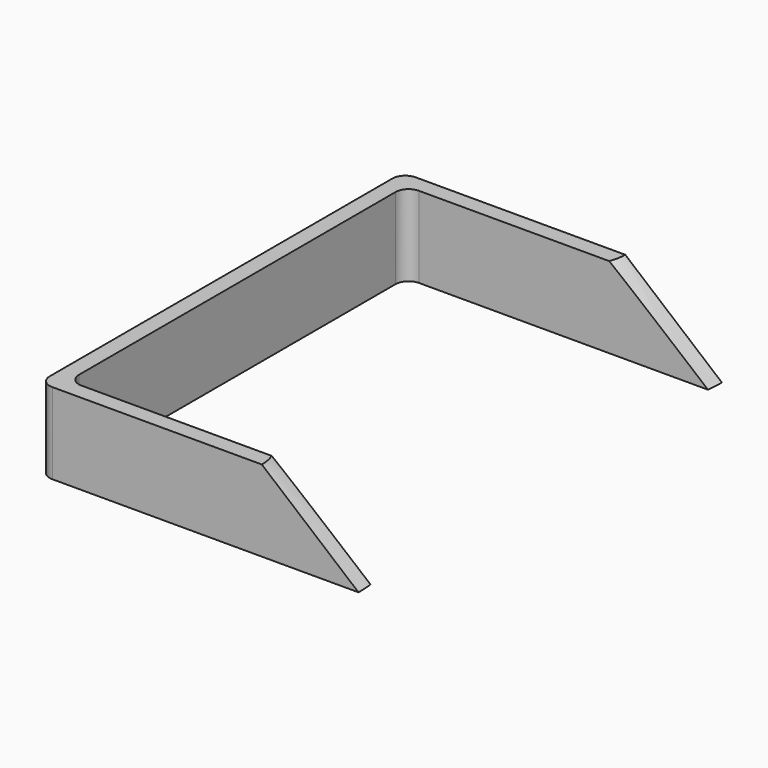
from build123d import *

# Parameters (mm, degrees)
F1_DEPTH     = 3.175
F2_DEPTH     = 19.05
F3_DEPTH     = 3.175
F4_T4_ANGLE  = 359.64
F4_T11_ANGLE = 359.64
F4_T16_ANGLE = 359.64
F4_T18_ANGLE = 359.64
F5_R         = 2.54
F6_W         = 173.444584012
F6_H         = 315.2023479342
F7_DEPTH     = 3.175


# Not quite as in the source:
# - a fillet or chamfer that OpenCascade refuses, or shapes differently, is made with other operations: its cross-section is extruded or revolved along the edge and cut away or added


with BuildPart() as f1:
    # F0 (on Top) → F1 (new body)
    with BuildSketch(Plane.XY):
        with BuildLine():
            Line((-34.925, 44.45), (-28.575, 44.45))
            ThreePointArc((-28.575, 44.45), (-39.4151280605, 48.9401280605), (-34.925, 38.1))
            Line((-34.925, 38.1), (-34.925, 44.45))
        make_face()
        with BuildLine():
            ThreePointArc((6.35, 44.45), (0, 50.8), (-6.35, 44.45))
            Line((-6.35, 44.45), (6.35, 44.45))
        make_face()
        with BuildLine():
            Line((-34.925, -44.45), (-34.925, -38.1))
            ThreePointArc((-34.925, -38.1), (-39.4151280605, -48.9401280605), (-28.575, -44.45))
            Line((-28.575, -44.45), (-34.925, -44.45))
        make_face()
        with BuildLine():
            Line((6.35, -44.45), (-6.35, -44.45))
            ThreePointArc((-6.35, -44.45), (0, -50.8), (6.35, -44.45))
        make_face()
        with BuildLine():
            ThreePointArc((-28.575, 44.45), (-28.7913710031, 42.8064990636), (-29.425738686, 41.275))
            Line((-29.425738686, 41.275), (-5.499261314, 41.275))
            ThreePointArc((-5.499261314, 41.275), (-6.1336289969, 42.8064990636), (-6.35, 44.45))
            Line((-6.35, 44.45), (-28.575, 44.45))
        make_face()
        with BuildLine():
            Line((-5.499261314, -41.275), (-29.425738686, -41.275))
            ThreePointArc((-29.425738686, -41.275), (-28.7913710031, -42.8064990636), (-28.575, -44.45))
            Line((-28.575, -44.45), (-6.35, -44.45))
            ThreePointArc((-6.35, -44.45), (-6.1336289969, -42.8064990636), (-5.499261314, -41.275))
        make_face()
        with BuildLine():
            Line((-31.75, -38.950738686), (-31.75, 38.950738686))
            ThreePointArc((-31.75, 38.950738686), (-33.2814990636, 38.3163710031), (-34.925, 38.1))
            Line((-34.925, 38.1), (-34.925, -38.1))
            ThreePointArc((-34.925, -38.1), (-33.2814990636, -38.3163710031), (-31.75, -38.950738686))
        make_face()
        with BuildLine():
            Line((-31.75, 38.950738686), (-31.75, 41.275))
            Line((-31.75, 41.275), (-29.425738686, 41.275))
            ThreePointArc((-29.425738686, 41.275), (-28.7913710031, 42.8064990636), (-28.575, 44.45))
            Line((-28.575, 44.45), (-34.925, 44.45))
            Line((-34.925, 44.45), (-34.925, 38.1))
            ThreePointArc((-34.925, 38.1), (-33.2814990636, 38.3163710031), (-31.75, 38.950738686))
        make_face()
        with BuildLine():
            ThreePointArc((-6.35, 44.45), (-6.1336289969, 42.8064990636), (-5.499261314, 41.275))
            Line((-5.499261314, 41.275), (5.499261314, 41.275))
            ThreePointArc((5.499261314, 41.275), (6.1336289969, 42.8064990636), (6.35, 44.45))
            Line((6.35, 44.45), (-6.35, 44.45))
        make_face()
        with BuildLine():
            Line((-31.75, -41.275), (-31.75, -38.950738686))
            ThreePointArc((-31.75, -38.950738686), (-33.2814990636, -38.3163710031), (-34.925, -38.1))
            Line((-34.925, -38.1), (-34.925, -44.45))
            Line((-34.925, -44.45), (-28.575, -44.45))
            ThreePointArc((-28.575, -44.45), (-28.7913710031, -42.8064990636), (-29.425738686, -41.275))
            Line((-29.425738686, -41.275), (-31.75, -41.275))
        make_face()
        with BuildLine():
            Line((5.499261314, -41.275), (-5.499261314, -41.275))
            ThreePointArc((-5.499261314, -41.275), (-6.1336289969, -42.8064990636), (-6.35, -44.45))
            Line((-6.35, -44.45), (6.35, -44.45))
            ThreePointArc((6.35, -44.45), (6.1336289969, -42.8064990636), (5.499261314, -41.275))
        make_face()
    extrude(amount=F1_DEPTH)

    # F0 (on Top) → F2 (join)
    with BuildSketch(Plane.XY):
        with BuildLine():
            ThreePointArc((-28.575, 44.45), (-28.7913710031, 42.8064990636), (-29.425738686, 41.275))
            Line((-29.425738686, 41.275), (-5.499261314, 41.275))
            ThreePointArc((-5.499261314, 41.275), (-6.1336289969, 42.8064990636), (-6.35, 44.45))
            Line((-6.35, 44.45), (-28.575, 44.45))
        make_face()
        with BuildLine():
            ThreePointArc((-6.35, 44.45), (-6.1336289969, 42.8064990636), (-5.499261314, 41.275))
            Line((-5.499261314, 41.275), (5.499261314, 41.275))
            ThreePointArc((5.499261314, 41.275), (6.1336289969, 42.8064990636), (6.35, 44.45))
            Line((6.35, 44.45), (-6.35, 44.45))
        make_face()
        with BuildLine():
            Line((-31.75, 38.950738686), (-31.75, 41.275))
            Line((-31.75, 41.275), (-29.425738686, 41.275))
            ThreePointArc((-29.425738686, 41.275), (-28.7913710031, 42.8064990636), (-28.575, 44.45))
            Line((-28.575, 44.45), (-34.925, 44.45))
            Line((-34.925, 44.45), (-34.925, 38.1))
            ThreePointArc((-34.925, 38.1), (-33.2814990636, 38.3163710031), (-31.75, 38.950738686))
        make_face()
        with BuildLine():
            Line((-31.75, -38.950738686), (-31.75, 38.950738686))
            ThreePointArc((-31.75, 38.950738686), (-33.2814990636, 38.3163710031), (-34.925, 38.1))
            Line((-34.925, 38.1), (-34.925, -38.1))
            ThreePointArc((-34.925, -38.1), (-33.2814990636, -38.3163710031), (-31.75, -38.950738686))
        make_face()
        with BuildLine():
            Line((-31.75, -41.275), (-31.75, -38.950738686))
            ThreePointArc((-31.75, -38.950738686), (-33.2814990636, -38.3163710031), (-34.925, -38.1))
            Line((-34.925, -38.1), (-34.925, -44.45))
            Line((-34.925, -44.45), (-28.575, -44.45))
            ThreePointArc((-28.575, -44.45), (-28.7913710031, -42.8064990636), (-29.425738686, -41.275))
            Line((-29.425738686, -41.275), (-31.75, -41.275))
        make_face()
        with BuildLine():
            Line((-5.499261314, -41.275), (-29.425738686, -41.275))
            ThreePointArc((-29.425738686, -41.275), (-28.7913710031, -42.8064990636), (-28.575, -44.45))
            Line((-28.575, -44.45), (-6.35, -44.45))
            ThreePointArc((-6.35, -44.45), (-6.1336289969, -42.8064990636), (-5.499261314, -41.275))
        make_face()
        with BuildLine():
            Line((5.499261314, -41.275), (-5.499261314, -41.275))
            ThreePointArc((-5.499261314, -41.275), (-6.1336289969, -42.8064990636), (-6.35, -44.45))
            Line((-6.35, -44.45), (6.35, -44.45))
            ThreePointArc((6.35, -44.45), (6.1336289969, -42.8064990636), (5.499261314, -41.275))
        make_face()
    extrude(amount=F2_DEPTH)

    # F0 (on Top) → F3 (join)
    with BuildSketch(Plane.XY):
        with BuildLine():
            ThreePointArc((6.35, 44.45), (6.1336289969, 42.8064990636), (5.499261314, 41.275))
            Line((5.499261314, 41.275), (31.75, 41.275))
            Line((31.75, 41.275), (31.75, -41.275))
            Line((31.75, -41.275), (5.499261314, -41.275))
            ThreePointArc((5.499261314, -41.275), (6.1336289969, -42.8064990636), (6.35, -44.45))
            Line((6.35, -44.45), (34.925, -44.45))
            Line((34.925, -44.45), (34.925, 44.45))
            Line((34.925, 44.45), (6.35, 44.45))
        make_face()
        with BuildLine():
            Line((-5.499261314, 41.275), (-29.425738686, 41.275))
            ThreePointArc((-29.425738686, 41.275), (-30.4348719395, 39.9598719395), (-31.75, 38.950738686))
            Line((-31.75, 38.950738686), (-31.75, -38.950738686))
            ThreePointArc((-31.75, -38.950738686), (-30.4348719395, -39.9598719395), (-29.425738686, -41.275))
            Line((-29.425738686, -41.275), (-5.499261314, -41.275))
            ThreePointArc((-5.499261314, -41.275), (0, -38.1), (5.499261314, -41.275))
            Line((5.499261314, -41.275), (31.75, -41.275))
            Line((31.75, -41.275), (31.75, 41.275))
            Line((31.75, 41.275), (5.499261314, 41.275))
            ThreePointArc((5.499261314, 41.275), (0, 38.1), (-5.499261314, 41.275))
        make_face()
        with BuildLine():
            Line((5.499261314, 41.275), (-5.499261314, 41.275))
            ThreePointArc((-5.499261314, 41.275), (0, 38.1), (5.499261314, 41.275))
        make_face()
        with BuildLine():
            Line((-29.425738686, 41.275), (-31.75, 41.275))
            Line((-31.75, 41.275), (-31.75, 38.950738686))
            ThreePointArc((-31.75, 38.950738686), (-30.4348719395, 39.9598719395), (-29.425738686, 41.275))
        make_face()
        with BuildLine():
            ThreePointArc((5.499261314, -41.275), (0, -38.1), (-5.499261314, -41.275))
            Line((-5.499261314, -41.275), (5.499261314, -41.275))
        make_face()
        with BuildLine():
            ThreePointArc((-29.425738686, -41.275), (-30.4348719395, -39.9598719395), (-31.75, -38.950738686))
            Line((-31.75, -38.950738686), (-31.75, -41.275))
            Line((-31.75, -41.275), (-29.425738686, -41.275))
        make_face()
    extrude(amount=F3_DEPTH)

    # F4: chamfer of 17.78 x 21.1893788763 on 4 edges, made by hand


with BuildPart() as f4_tool2:
    # F4_s3 → F4_t4 (revolve)
    with BuildSketch(Plane(origin=(-7.9045602021, -1.4531788711, 0), x_dir=(0, 0, 1), z_dir=(-0.983517952, -0.1808105031, 0))):
        Polygon((3.175, -16.1779940912), (20.955, -37.3673729675), (3.175, -37.3673729675), align=None)
    revolve(axis=Axis((0, -44.45, 3.175), (0, 0, -1)), revolution_arc=F4_T4_ANGLE)

    split(bisect_by=Plane.XY.offset(19.05), keep=Keep.BOTTOM)

    split(bisect_by=Plane.XZ.offset(44.45), keep=Keep.BOTTOM)

    split(bisect_by=Plane.XZ.offset(41.275), keep=Keep.TOP)


with BuildPart() as f1_1:
    add(f1.part)

    # F4_t1: union F4_tool2
    add(f4_tool2.part)


with BuildPart() as f4_tool9:
    # F4_s10 → F4_t11 (revolve)
    with BuildSketch(Plane(origin=(-8.164955624, 1.5541479455, 0), x_dir=(0, 0, 1), z_dir=(0.9823624798, -0.186986519, 0))):
        Polygon((20.955, -37.3160122271), (3.175, -16.1266333508), (3.175, -37.3160122271), align=None)
    revolve(axis=Axis((0, 44.45, 3.175), (0, 0, -1)), revolution_arc=F4_T11_ANGLE)

    split(bisect_by=Plane.XZ.offset(-44.45), keep=Keep.TOP)

    split(bisect_by=Plane.XY.offset(19.05), keep=Keep.BOTTOM)

    split(bisect_by=Plane.XZ.offset(-41.275), keep=Keep.BOTTOM)


with BuildPart() as f1_2:
    add(f1_1.part)

    # F4_t8: union F4_tool9
    add(f4_tool9.part)

    # F4_s15 → F4_t16 (revolve, cut)
    with BuildSketch(Plane(origin=(-0.1396428746, -0.0004387025, 0), x_dir=(0, 0, 1), z_dir=(0.9999950652, 0.0031415875, 0))):
        Polygon((-14.605, 38.0997806482), (-9.276717342, 44.4497806482), (3.175, 44.4497806482), (3.175, 38.0997806482), align=None)
    revolve(axis=Axis((0, -44.45, 3.175), (0, 0, 1)), revolution_arc=F4_T16_ANGLE, mode=Mode.SUBTRACT)

    # F4_s17 → F4_t18 (revolve, cut)
    with BuildSketch(Plane(origin=(0.1396428746, 0.0004387025, 0), x_dir=(0, 0, 1), z_dir=(-0.9999950652, -0.0031415875, 0))):
        Polygon((-14.605, 38.0997806482), (-9.276717342, 44.4497806482), (3.175, 44.4497806482), (3.175, 38.0997806482), align=None)
    revolve(axis=Axis((0, 44.45, 3.175), (0, 0, 1)), revolution_arc=F4_T18_ANGLE, mode=Mode.SUBTRACT)

    # F5
    f5_edges = [f1_2.edges().sort_by_distance(p)[0] for p in [
        (-31.75, 41.275, 11.1125),
        (-31.75, -41.275, 11.1125),
        (-34.925, -44.45, 11.1125),
        (-34.925, 44.45, 11.1125),
    ]]
    fillet(f5_edges, radius=F5_R)

    # F6 (on Top) → F7 (cut)
    with BuildSketch(Plane.XY):
        with Locations((-10.1288706064, 37.9523970187)):
            Rectangle(F6_W, F6_H)
    extrude(amount=F7_DEPTH, mode=Mode.SUBTRACT)


solid = f1_2.part
